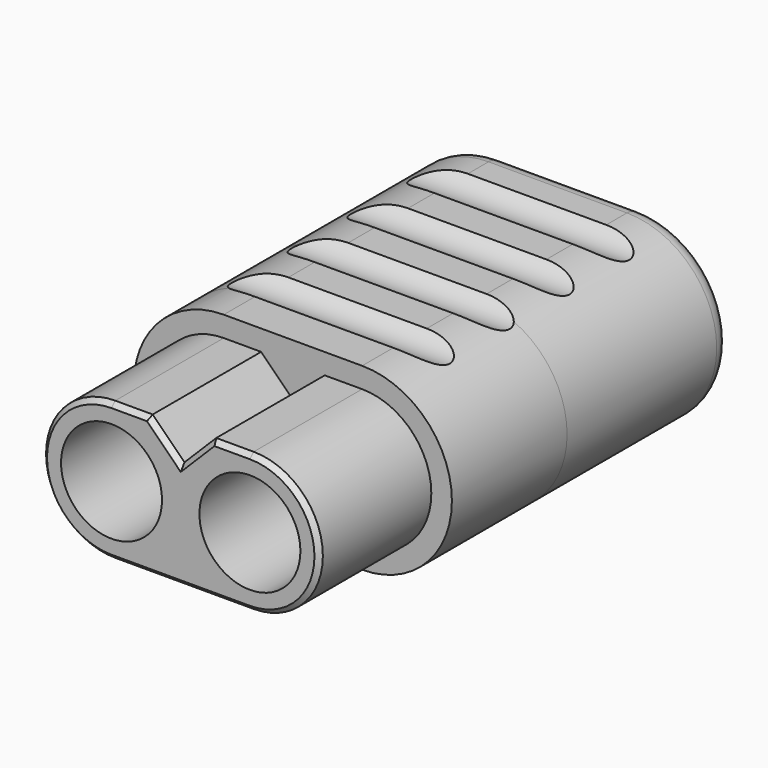
from build123d import *

# Parameters (mm, degrees)
F0_R      = 2.8
F1_DEPTH  = 3
F0_R_2    = 2.425
F2_DEPTH  = 2.2
F3_R      = 2.7
F4_DEPTH  = 2.5
F5_R      = 2.7
F6_DEPTH  = 7.5
F7_R      = 3.2
F8_DEPTH  = 11
F9_R      = 1
F10_SIZE  = 0.25
F11_R     = 1.5
F12_DEPTH = 8.5


# Not quite as in the source:
# - a feature names something its author has since deleted; it is built from what else it names


with BuildPart() as f1:
    # F0 (on Front) → F1 (new body)
    with BuildSketch(Plane.XZ):
        with BuildLine():
            Line((0, 4.8), (-3.7, 4.8))
            ThreePointArc((-3.7, 4.8), (-7.0941125497, 3.3941125497), (-8.5, 0))
            ThreePointArc((-8.5, 0), (-7.0941125497, -3.3941125497), (-3.7, -4.8))
            Line((-3.7, -4.8), (0, -4.8))
            Line((0, -4.8), (3.7, -4.8))
            ThreePointArc((3.7, -4.8), (7.0941125497, -3.3941125497), (8.5, 0))
            ThreePointArc((8.5, 0), (7.0941125497, 3.3941125497), (3.7, 4.8))
            Line((3.7, 4.8), (0, 4.8))
        make_face()
        with Locations((-3.7, 0)):
            Circle(F0_R, mode=Mode.SUBTRACT)
        with Locations((3.7, 0)):
            Circle(F0_R, mode=Mode.SUBTRACT)
    extrude(amount=-F1_DEPTH)

    # F0 (on Front) → F2 (join)
    with BuildSketch(Plane.XZ):
        with BuildLine():
            Line((0, 4.8), (-3.7, 4.8))
            ThreePointArc((-3.7, 4.8), (-7.0941125497, 3.3941125497), (-8.5, 0))
            ThreePointArc((-8.5, 0), (-7.0941125497, -3.3941125497), (-3.7, -4.8))
            Line((-3.7, -4.8), (0, -4.8))
            Line((0, -4.8), (3.7, -4.8))
            ThreePointArc((3.7, -4.8), (7.0941125497, -3.3941125497), (8.5, 0))
            ThreePointArc((8.5, 0), (7.0941125497, 3.3941125497), (3.7, 4.8))
            Line((3.7, 4.8), (0, 4.8))
        make_face()
        with Locations((-3.7, 0)):
            Circle(F0_R, mode=Mode.SUBTRACT)
        with Locations((3.7, 0)):
            Circle(F0_R, mode=Mode.SUBTRACT)
        with Locations((-3.7, 0)):
            Circle(F0_R)
        with Locations((-3.7, 0)):
            Circle(F0_R_2, mode=Mode.SUBTRACT)
        with Locations((3.7, 0)):
            Circle(F0_R)
        with Locations((3.7, 0)):
            Circle(F0_R_2, mode=Mode.SUBTRACT)
    extrude(amount=F2_DEPTH)

    # F3 (on face) → F4 (join)
    with BuildSketch(Plane.XZ.offset(2.2)):
        with BuildLine():
            ThreePointArc((3.7, -4.8), (8.5, 0), (3.7, 4.8))
            Line((3.7, 4.8), (-3.7, 4.8))
            ThreePointArc((-3.7, 4.8), (-8.5, 0), (-3.7, -4.8))
            Line((-3.7, -4.8), (3.7, -4.8))
        make_face()
        with Locations((-3.7, 0)):
            Circle(F3_R, mode=Mode.SUBTRACT)
        with Locations((3.7, 0)):
            Circle(F3_R, mode=Mode.SUBTRACT)
    extrude(amount=F4_DEPTH)

    # F5 (on face) → F6 (join)
    with BuildSketch(Plane.XZ.offset(4.7)):
        with BuildLine():
            ThreePointArc((-3.7, 3.7), (-7.4, 0), (-3.7, -3.7))
            Line((-3.7, -3.7), (0, -3.7))
            Line((0, -3.7), (3.7, -3.7))
            ThreePointArc((3.7, -3.7), (7.4, 0), (3.7, 3.7))
            Line((3.7, 3.7), (1.7, 3.7))
            Line((1.7, 3.7), (0, 2))
            Line((0, 2), (-1.7, 3.7))
            Line((-1.7, 3.7), (-3.7, 3.7))
        make_face()
        with Locations((-3.7, 0)):
            Circle(F5_R, mode=Mode.SUBTRACT)
        with Locations((3.7, 0)):
            Circle(F5_R, mode=Mode.SUBTRACT)
    extrude(amount=F6_DEPTH)

    # F7 (on face) → F8 (join)
    with BuildSketch(Plane(origin=(0, 3, 0), x_dir=(-1, 0, 0), z_dir=(0, 1, 0))):
        with BuildLine():
            ThreePointArc((3.7, -4.8), (8.5, 0), (3.7, 4.8))
            Line((3.7, 4.8), (-3.7, 4.8))
            ThreePointArc((-3.7, 4.8), (-8.5, 0), (-3.7, -4.8))
            Line((-3.7, -4.8), (3.7, -4.8))
        make_face()
        with Locations((-3.7, 0)):
            Circle(F7_R, mode=Mode.SUBTRACT)
        with Locations((3.7, 0)):
            Circle(F7_R, mode=Mode.SUBTRACT)
    extrude(amount=F8_DEPTH)

    # F9
    f9_edges = [f1.edges().sort_by_distance(p)[0] for p in [
        (0, 14, 4.8),
    ]]
    fillet(f9_edges, radius=F9_R)

    # F10
    f10_edges = [f1.edges().sort_by_distance(p)[0] for p in [
        (-2.7, -12.2, 3.7),
        (-0.85, -12.2, 2.85),
        (0.85, -12.2, 2.85),
    ]]
    chamfer(f10_edges, length=F10_SIZE)

    # F11 (on Right) → F12 (cut, symmetric)
    with BuildSketch(Plane.YZ):
        with Locations((6.5, 5.8)):
            Circle(F11_R)
        with Locations((2.5, 5.8)):
            Circle(F11_R)
        with Locations((2.5, -5.8)):
            Circle(F11_R)
        with Locations((6.5, -5.8)):
            Circle(F11_R)
        with Locations((10.5, -5.8)):
            Circle(F11_R)
        with Locations((10.5, 5.8)):
            Circle(F11_R)
        with Locations((-1.5, 5.8)):
            Circle(F11_R)
        with Locations((-1.5, -5.8)):
            Circle(F11_R)
    extrude(amount=F12_DEPTH, both=True, mode=Mode.SUBTRACT)


solid = f1.part
